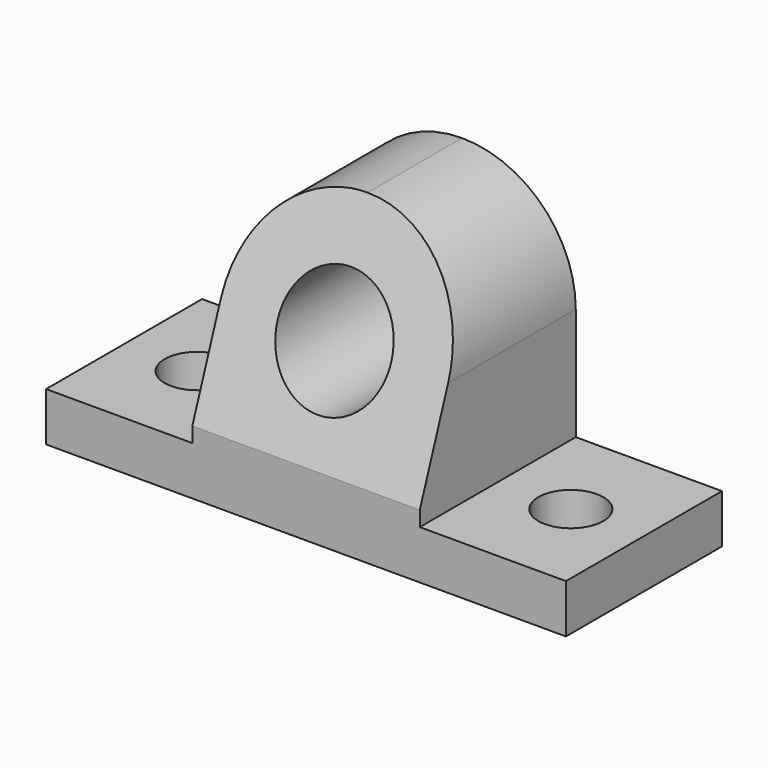
from build123d import *

# Parameters (mm, degrees)
F0_W          = 160
F0_H          = 60
F0_R          = 10
F1_DEPTH      = 15
F3_DEPTH      = 30
F3_DEPTH_BACK = 30
F4_T1_DEPTH   = 407.2453152316
F5_R          = 34.99999


# Not quite as in the source:
# - a fillet or chamfer that OpenCascade refuses, or shapes differently, is made with other operations: its cross-section is extruded or revolved along the edge and cut away or added
# - a fillet or chamfer is up to 0.001 mm smaller than in the source, because OpenCascade refuses the exact size


with BuildPart() as f1:
    # F0 (on Top) → F1 (new body)
    with BuildSketch(Plane.XY):
        Rectangle(F0_W, F0_H)
        with Locations((-57.5, 0)):
            Circle(F0_R, mode=Mode.SUBTRACT)
        with Locations((57.5, 0)):
            Circle(F0_R, mode=Mode.SUBTRACT)
    extrude(amount=F1_DEPTH)

    # F2 (on Front) → F3 (join, two sides)
    with BuildSketch(Plane.XZ) as f3_sk:
        with BuildLine():
            Line((35.0165497145, 49.646243304), (17.5165497145, 49.646243304))
            ThreePointArc((17.5165497145, 49.646243304), (0.0165497145, 32.146243304), (-17.4834502855, 49.646243304))
            Line((-17.4834502855, 49.646243304), (-34.9834502855, 49.646243304))
            Line((-34.9834502855, 49.646243304), (-34.9834502855, 14.646243304))
            Line((-34.9834502855, 14.646243304), (35.0165497145, 14.646243304))
            Line((35.0165497145, 14.646243304), (35.0165497145, 49.646243304))
        make_face()
        with BuildLine():
            ThreePointArc((-17.4834502855, 49.646243304), (0.0165497145, 67.146243304), (17.5165497145, 49.646243304))
            Line((17.5165497145, 49.646243304), (35.0165497145, 49.646243304))
            Line((35.0165497145, 49.646243304), (35.0165497145, 54.9693842517))
            Line((35.0165497145, 54.9693842517), (35.0165497145, 84.646243304))
            Line((35.0165497145, 84.646243304), (-34.9834502855, 84.646243304))
            Line((-34.9834502855, 84.646243304), (-34.9834502855, 49.646243304))
            Line((-34.9834502855, 49.646243304), (-17.4834502855, 49.646243304))
        make_face()
    extrude(amount=F3_DEPTH)
    extrude(f3_sk.sketch, amount=-F3_DEPTH_BACK)

    # F4: chamfer of 65 x 23.6580652273 on 1 edges, made by hand

    # F4_s2 → F4_t1 (cut)
    with BuildSketch(Plane.YZ.offset(-203.6061079013)):
        Polygon((-30, 19.646243304), (-6.3419347727, 84.646243304), (-30, 84.646243304), align=None)
    extrude(amount=F4_T1_DEPTH, mode=Mode.SUBTRACT)

    # F5 (radius 35 in the source; OpenCascade refuses exactly that, so slightly less here)
    f5_edges = [f1.edges().sort_by_distance(p)[0] for p in [
        (35.01655, 11.829033, 84.646243),
        (-34.98345, 11.829033, 84.646243),
    ]]
    fillet(f5_edges, radius=F5_R)


solid = f1.part
